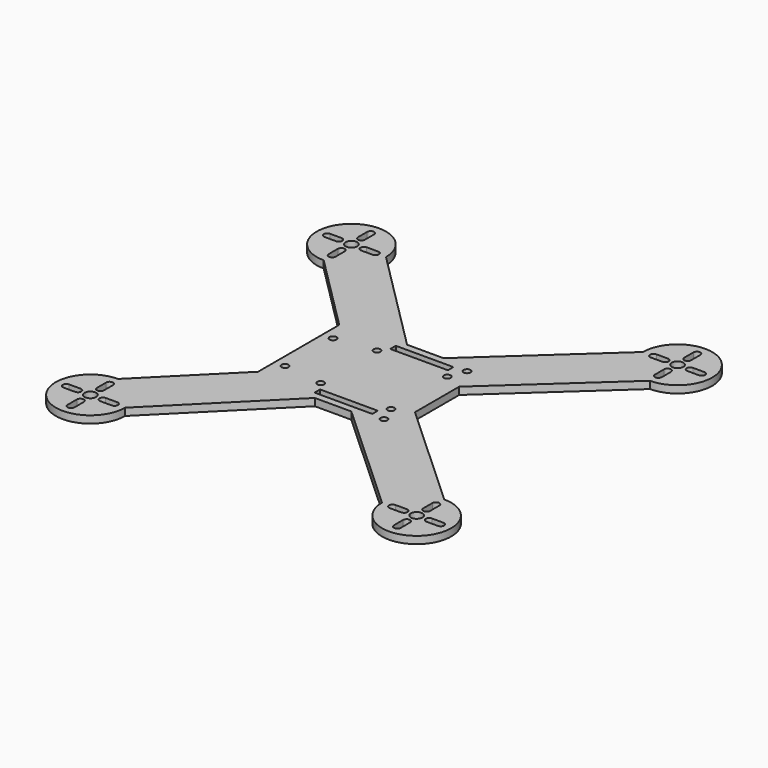
from build123d import *

# Parameters (mm, degrees)
F0_R     = 2.5
F0_R_2   = 1.5
F0_W     = 25
F0_H     = 3
F1_DEPTH = 3.175


# Not quite as in the source:
# - ends of sketch curves that miss each other by under 0.0002 mm in the source are joined


with BuildPart() as f1:
    # F0 (on Top) → F1 (new body)
    with BuildSketch(Plane.XY):
        with BuildLine():
            Line((-10.0000000587, 25), (-55.7106781187, 70.7106779065))
            ThreePointArc((-55.7106781187, 70.7106779065), (-81.3172799026, 81.3172797703), (-70.7106779065, 55.7106781187))
            Line((-70.7106779065, 55.7106781187), (-37, 22.0000003253))
            Line((-37, 22.0000003253), (-37, -22.0000003253))
            Line((-37, -22.0000003253), (-70.7106779065, -55.7106781187))
            ThreePointArc((-70.7106779065, -55.7106781187), (-81.3172798365, -81.3172798365), (-55.7106781187, -70.7106779065))
            Line((-55.7106781187, -70.7106779065), (-10.0000000587, -25))
            Line((-10.0000000587, -25), (5.8262266936, -25))
            Line((5.8262266936, -25), (55.7106781187, -70.7106780935))
            ThreePointArc((55.7106781187, -70.7106780935), (81.3172798365, -81.3172798365), (70.7106780935, -55.7106781187))
            Line((70.7106780935, -55.7106781187), (23, -11.9918965954))
            Line((23, -11.9918965954), (23, 11.9918965954))
            Line((23, 11.9918965954), (70.7106780935, 55.7106781187))
            ThreePointArc((70.7106780935, 55.7106781187), (81.3172798365, 81.3172798365), (55.7106781187, 70.7106779065))
            Line((55.7106781187, 70.7106779065), (5.8262266936, 25))
            Line((5.8262266936, 25), (-10.0000000587, 25))
        make_face()
        with BuildLine():
            Line((-72.210678, -81.1510407925), (-72.210678, -76.1510407925))
            ThreePointArc((-72.210678, -76.1510407925), (-70.710678, -74.6510407925), (-69.210678, -76.1510407925))
            Line((-69.210678, -76.1510407925), (-69.210678, -81.1510407925))
            ThreePointArc((-69.210678, -81.1510407925), (-70.710678, -82.6510407925), (-72.210678, -81.1510407925))
        make_face(mode=Mode.SUBTRACT)
        with BuildLine():
            Line((-81.1510407874, -69.2106756767), (-76.1510407874, -69.2106756935))
            ThreePointArc((-76.1510407874, -69.2106756935), (-74.6510407925, -70.7106782241), (-76.1510407975, -72.2106782191))
            Line((-76.1510407975, -72.2106782191), (-81.1510407975, -72.2106755673))
            ThreePointArc((-81.1510407975, -72.2106755673), (-82.6510407925, -70.7106781972), (-81.1510407874, -69.2106756767))
        make_face(mode=Mode.SUBTRACT)
        with Locations((-70.7106781187, -70.7106781187)):
            Circle(F0_R, mode=Mode.SUBTRACT)
        with BuildLine():
            Line((-60.2703154499, -72.210678035), (-65.2703154499, -72.2106780183))
            ThreePointArc((-65.2703154499, -72.2106780183), (-66.7703154448, -70.7106780132), (-65.2703154398, -69.2106780183))
            Line((-65.2703154398, -69.2106780183), (-60.2703154398, -69.210678035))
            ThreePointArc((-60.2703154398, -69.210678035), (-58.7703154448, -70.7106780401), (-60.2703154499, -72.210678035))
        make_face(mode=Mode.SUBTRACT)
        with BuildLine():
            Line((-69.210678035, -60.2703154398), (-69.2106780183, -65.2703154398))
            ThreePointArc((-69.2106780183, -65.2703154398), (-70.7106780132, -66.7703154448), (-72.2106780183, -65.2703154499))
            Line((-72.2106780183, -65.2703154499), (-72.210678035, -60.2703154499))
            ThreePointArc((-72.210678035, -60.2703154499), (-70.7106780401, -58.7703154448), (-69.210678035, -60.2703154398))
        make_face(mode=Mode.SUBTRACT)
        with Locations((-32.5, -13)):
            Circle(F0_R_2, mode=Mode.SUBTRACT)
        with Locations((-15.25, -15.25)):
            Circle(F0_R_2, mode=Mode.SUBTRACT)
        with BuildLine():
            Line((60.2703154398, -69.210678035), (65.2703154398, -69.2106780183))
            ThreePointArc((65.2703154398, -69.2106780183), (66.7703154448, -70.7106780132), (65.2703154499, -72.2106780183))
            Line((65.2703154499, -72.2106780183), (60.2703154499, -72.210678035))
            ThreePointArc((60.2703154499, -72.210678035), (58.7703154448, -70.7106780401), (60.2703154398, -69.210678035))
        make_face(mode=Mode.SUBTRACT)
        with BuildLine():
            ThreePointArc((69.210678, -76.1510407925), (70.710678, -74.6510407925), (72.210678, -76.1510407925))
            Line((72.210678, -76.1510407925), (72.210678, -81.1510407925))
            ThreePointArc((72.210678, -81.1510407925), (70.710678, -82.6510407925), (69.210678, -81.1510407925))
            Line((69.210678, -81.1510407925), (69.210678, -76.1510407925))
        make_face(mode=Mode.SUBTRACT)
        with Locations((70.7106781187, -70.7106781187)):
            Circle(F0_R, mode=Mode.SUBTRACT)
        with BuildLine():
            ThreePointArc((76.1510407975, -72.2106782191), (74.6510407925, -70.7106782241), (76.1510407874, -69.2106782191))
            Line((76.1510407874, -69.2106782191), (81.1510407874, -69.2106756767))
            ThreePointArc((81.1510407874, -69.2106756767), (82.6510407925, -70.7106781972), (81.1510407975, -72.2106782023))
            Line((81.1510407975, -72.2106782023), (76.1510407975, -72.2106782191))
        make_face(mode=Mode.SUBTRACT)
        with BuildLine():
            ThreePointArc((72.2106780183, -65.2703154499), (70.7106780132, -66.7703154448), (69.2106780183, -65.2703154398))
            Line((69.2106780183, -65.2703154398), (69.210678035, -60.2703154398))
            ThreePointArc((69.210678035, -60.2703154398), (70.7106780401, -58.7703154448), (72.210678035, -60.2703154499))
            Line((72.210678035, -60.2703154499), (72.2106780183, -65.2703154499))
        make_face(mode=Mode.SUBTRACT)
        with Locations((18, -22.5)):
            Circle(F0_R_2, mode=Mode.SUBTRACT)
        with Locations((0, -20.5)):
            Rectangle(F0_W, F0_H, mode=Mode.SUBTRACT)
        with Locations((15.25, -15.25)):
            Circle(F0_R_2, mode=Mode.SUBTRACT)
        with Locations((-32.5, 13)):
            Circle(F0_R_2, mode=Mode.SUBTRACT)
        with Locations((-15.25, 15.25)):
            Circle(F0_R_2, mode=Mode.SUBTRACT)
        with BuildLine():
            ThreePointArc((-72.2106780183, 65.2703154499), (-70.7106780132, 66.7703154448), (-69.2106780183, 65.2703154398))
            Line((-69.2106780183, 65.2703154398), (-69.210678035, 60.2703154398))
            ThreePointArc((-69.210678035, 60.2703154398), (-70.7106780401, 58.7703154448), (-72.210678035, 60.2703154499))
            Line((-72.210678035, 60.2703154499), (-72.2106780183, 65.2703154499))
        make_face(mode=Mode.SUBTRACT)
        with BuildLine():
            ThreePointArc((-76.1510407975, 72.2106782191), (-74.6510407925, 70.7106782241), (-76.1510407874, 69.2106782191))
            Line((-76.1510407874, 69.2106782191), (-81.1510407874, 69.2106782023))
            ThreePointArc((-81.1510407874, 69.2106782023), (-82.6510407925, 70.7106781972), (-81.1510407975, 72.2106782023))
            Line((-81.1510407975, 72.2106782023), (-76.1510407975, 72.2106782191))
        make_face(mode=Mode.SUBTRACT)
        with BuildLine():
            ThreePointArc((-68.9429111657, 72.4784450716), (-68.4009792874, 71.6673866996), (-68.2106781187, 70.7106781187))
            ThreePointArc((-68.2106781187, 70.7106781187), (-69.7539695377, 68.4009792874), (-72.4784450716, 68.9429111657))
            ThreePointArc((-72.4784450716, 68.9429111657), (-72.4784450716, 72.4784450716), (-68.9429111657, 72.4784450716))
        make_face(mode=Mode.SUBTRACT)
        with BuildLine():
            Line((-69.210678, 81.1510407925), (-69.210678, 76.1510407925))
            ThreePointArc((-69.210678, 76.1510407925), (-70.710678, 74.6510407925), (-72.210678, 76.1510407925))
            Line((-72.210678, 76.1510407925), (-72.210678, 81.1510407925))
            ThreePointArc((-72.210678, 81.1510407925), (-70.710678, 82.6510407925), (-69.210678, 81.1510407925))
        make_face(mode=Mode.SUBTRACT)
        with BuildLine():
            Line((-60.2703154398, 69.2106755095), (-65.2703154398, 69.2106754927))
            ThreePointArc((-65.2703154398, 69.2106754927), (-66.7703154448, 70.7106780132), (-65.2703154499, 72.2106780183))
            Line((-65.2703154499, 72.2106780183), (-60.2703154499, 72.2106754))
            ThreePointArc((-60.2703154499, 72.2106754), (-58.7703154448, 70.7106780401), (-60.2703154398, 69.2106755095))
        make_face(mode=Mode.SUBTRACT)
        with Locations((0, 20.5)):
            Rectangle(F0_W, F0_H, mode=Mode.SUBTRACT)
        with Locations((15.25, 15.25)):
            Circle(F0_R_2, mode=Mode.SUBTRACT)
        with Locations((18, 22.5)):
            Circle(F0_R_2, mode=Mode.SUBTRACT)
        with BuildLine():
            Line((69.210678035, 60.2703154398), (69.2106780183, 65.2703154398))
            ThreePointArc((69.2106780183, 65.2703154398), (70.7106780132, 66.7703154448), (72.2106780183, 65.2703154499))
            Line((72.2106780183, 65.2703154499), (72.210678035, 60.2703154499))
            ThreePointArc((72.210678035, 60.2703154499), (70.7106780401, 58.7703154448), (69.210678035, 60.2703154398))
        make_face(mode=Mode.SUBTRACT)
        with BuildLine():
            ThreePointArc((65.2703154499, 72.2106780183), (66.7703154448, 70.7106780132), (65.2703154398, 69.2106780183))
            Line((65.2703154398, 69.2106780183), (60.2703154398, 69.2106805606))
            ThreePointArc((60.2703154398, 69.2106805606), (58.7703154448, 70.7106780401), (60.2703154499, 72.210678035))
            Line((60.2703154499, 72.210678035), (65.2703154499, 72.2106780183))
        make_face(mode=Mode.SUBTRACT)
        with Locations((70.7106781187, 70.7106781187)):
            Circle(F0_R, mode=Mode.SUBTRACT)
        with BuildLine():
            Line((81.1510407874, 69.2106731512), (76.1510407874, 69.210673168))
            ThreePointArc((76.1510407874, 69.210673168), (74.6510407925, 70.7106782241), (76.1510407975, 72.2106782191))
            Line((76.1510407975, 72.2106782191), (81.1510407975, 72.2106729322))
            ThreePointArc((81.1510407975, 72.2106729322), (82.6510407925, 70.7106781972), (81.1510407874, 69.2106731512))
        make_face(mode=Mode.SUBTRACT)
        with BuildLine():
            Line((72.210678, 81.1510407925), (72.210678, 76.1510407925))
            ThreePointArc((72.210678, 76.1510407925), (70.710678, 74.6510407925), (69.210678, 76.1510407925))
            Line((69.210678, 76.1510407925), (69.210678, 81.1510407925))
            ThreePointArc((69.210678, 81.1510407925), (70.710678, 82.6510407925), (72.210678, 81.1510407925))
        make_face(mode=Mode.SUBTRACT)
    extrude(amount=F1_DEPTH)


solid = f1.part
